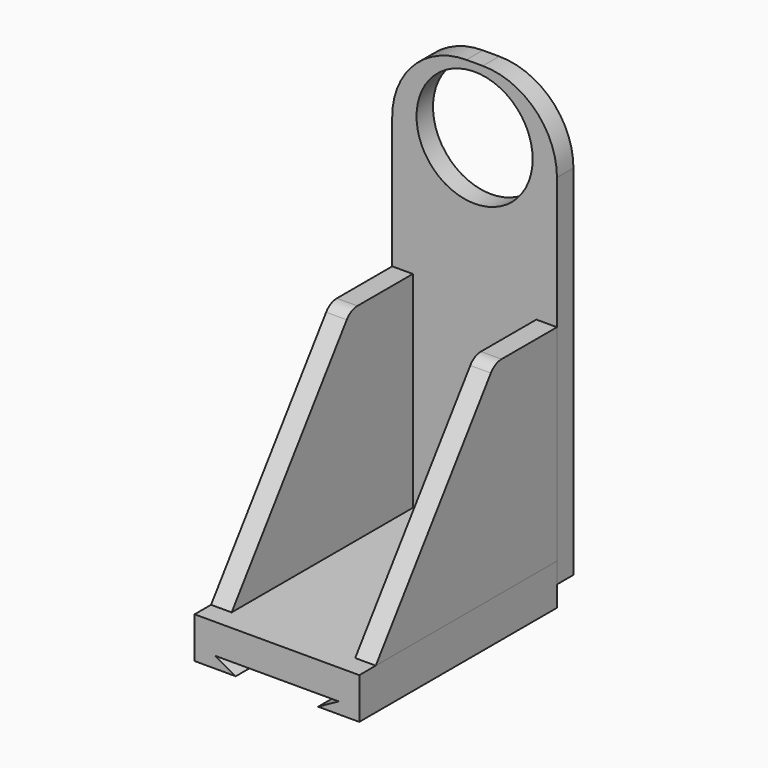
from build123d import *

# Parameters (mm, degrees)
F0_W      = 50.8
F0_H      = 76.2
F1_DEPTH  = 12.7
F2_W      = 50.8
F2_H      = 127
F2_H_2    = 6.35
F3_DEPTH  = 6.35
F5_DEPTH  = 6.35
F7_DEPTH  = 6.35
F8_R      = 5.08
F8_2_R    = 5.08
F9_R      = 17.907
F10_DEPTH = 25.4
F12_DEPTH = 82.55
F13_R     = 22.86
F14_R     = 7.239
F15_DEPTH = 82.551


# Not quite as in the source:
# - a feature names something its author has since deleted; it is built from what else it names


with BuildPart() as f1:
    # F0 (on Top) → F1 (new body)
    with BuildSketch(Plane.XY):
        Rectangle(F0_W, F0_H)
    extrude(amount=F1_DEPTH)

    # F11 (on face) → F12 (cut, through all)
    with BuildSketch(Plane.XZ.offset(38.1)):
        Polygon((-12.7, 0), (0, 0), (12.7, 0), (19.05, 3.5051606157), (-19.05, 3.5051606157), align=None)
    extrude(amount=-F12_DEPTH, mode=Mode.SUBTRACT)


with BuildPart() as f3:
    # F2 (on face) → F3 (new body)
    with BuildSketch(Plane(origin=(0, 38.1, 0), x_dir=(-1, 0, 0), z_dir=(0, 1, 0))):
        with Locations((0, 76.2)):
            Rectangle(F2_W, F2_H)
        with Locations((0, 9.525)):
            Rectangle(F2_W, F2_H_2)
    extrude(amount=F3_DEPTH)

    # F9 (on face) → F10 (cut)
    with BuildSketch(Plane.XZ.offset(-38.1)):
        with Locations((0, 119.38)):
            Circle(F9_R)
    extrude(amount=-F10_DEPTH, mode=Mode.SUBTRACT)

    # F13
    f13_edges = [f3.edges().sort_by_distance(p)[0] for p in [
        (25.4, 41.275, 139.7),
        (-25.4, 41.275, 139.7),
    ]]
    fillet(f13_edges, radius=F13_R)

    # F14 (on face) → F15 (cut, through all)
    with BuildSketch(Plane(origin=(0, 44.45, 0), x_dir=(-1, 0, 0), z_dir=(0, 1, 0))):
        with Locations((0, 25.4)):
            Circle(F14_R)
    extrude(amount=-F15_DEPTH, mode=Mode.SUBTRACT)


with BuildPart() as f5:
    # F4 (on face) → F5 (new body)
    with BuildSketch(Plane.YZ.offset(25.4)):
        Polygon((-31.75, 12.7), (38.1, 12.7), (38.1, 76.2), (14.1410465515, 76.2), align=None)
    extrude(amount=-F5_DEPTH)

    # F8#2
    f8_2_edges = [f5.edges().sort_by_distance(p)[0] for p in [
        (22.225, 14.141047, 76.2),
    ]]
    fillet(f8_2_edges, radius=F8_2_R)


with BuildPart() as f7:
    # F6 (on face) → F7 (new body)
    with BuildSketch(Plane(origin=(-25.4, 0, 0), x_dir=(0, -1, 0), z_dir=(-1, 0, 0))):
        Polygon((-38.1, 76.2), (-38.1, 12.7), (31.75, 12.7), (-14.1410465515, 76.2), align=None)
    extrude(amount=-F7_DEPTH)

    # F8
    f8_edges = [f7.edges().sort_by_distance(p)[0] for p in [
        (-22.225, 14.141047, 76.2),
    ]]
    fillet(f8_edges, radius=F8_R)


solid = Compound([f1.part, f3.part, f5.part, f7.part])
